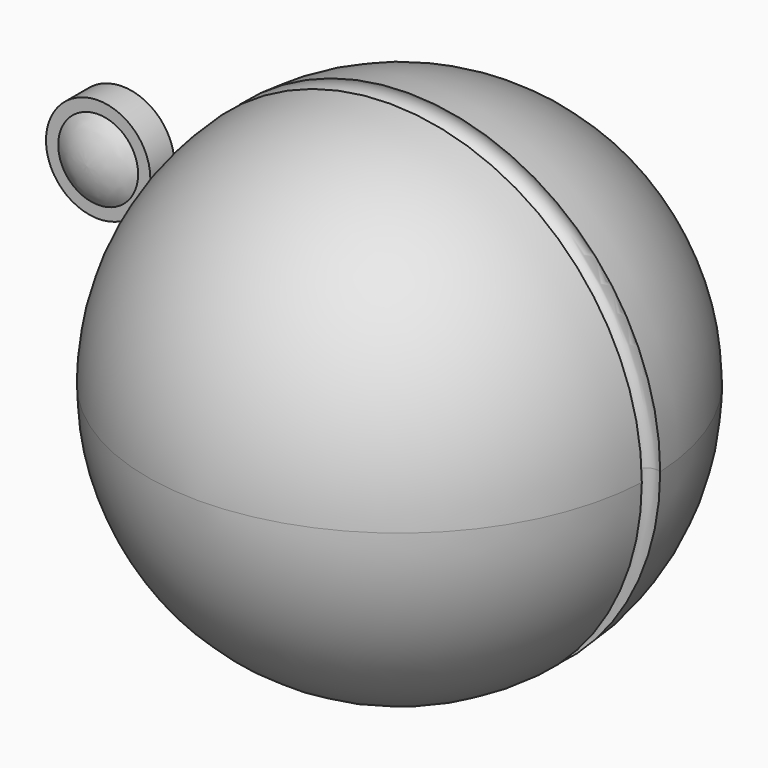
from build123d import *

# Parameters (mm, degrees)
F2_ANGLE  = 180
F5_R      = 7.25
F6_DEPTH  = 25
F8_W      = 26.5384614468
F8_H      = 20.0961548835
F9_DEPTH  = 20.8
F10_R     = 5.5512855598
F11_DEPTH = 2


# Not quite as in the source:
# - a fillet or chamfer that OpenCascade refuses, or shapes differently, is made with other operations: its cross-section is extruded or revolved along the edge and cut away or added


with BuildPart() as f2:
    # F0 (on Top) → F2 (revolve)
    with BuildSketch(Plane.XY):
        with BuildLine():
            Line((0, 30), (0, 35))
            ThreePointArc((0, 35), (-24.1771803229, 25.3073892694), (-34.9635036496, 1.5979400934))
            ThreePointArc((-34.9635036496, 1.5979400934), (-33.2976690142, 1.4681844889), (-32.5, 0))
            ThreePointArc((-32.5, 0), (-33.2976690142, -1.4681844889), (-34.9635036496, -1.5979400934))
            ThreePointArc((-34.9635036496, -1.5979400934), (-24.1771803229, -25.3073892694), (0, -35))
            Line((0, -35), (0, -30))
            ThreePointArc((0, -30), (-30, 0), (0, 30))
        make_face()
    revolve(axis=Axis((0, 0.055314973, 0), (0, -1, 0)), revolution_arc=F2_ANGLE)


with BuildPart() as f3_1:
    # F3: instance of F2
    add(f2.part.mirror(Plane.XY))


with BuildPart() as f6:
    # F5 (on Front) → F6 (new body)
    with BuildSketch(Plane.XZ):
        with Locations((-58.4951840291, 0)):
            Circle(F5_R)
    extrude(amount=-F6_DEPTH)

    # F4 (on Top) → F7 (revolve)
    with BuildSketch(Plane.XY):
        with BuildLine():
            Line((-58.4951840291, 24.5332963728), (-58.4951840291, 27.9332963728))
            ThreePointArc((-58.4951840291, 27.9332963728), (-60.1951840291, 26.2332963728), (-58.4951840291, 24.5332963728))
        make_face()
    revolve(axis=Axis((-58.4951840291, 26.2332963728, 0), (0, -1, 0)))

    # F8 (on Front) → F9 (cut)
    with BuildSketch(Plane.XZ):
        with Locations((-55.8634325862, -0.4141749814)):
            Rectangle(F8_W, F8_H)
    extrude(amount=-F9_DEPTH, mode=Mode.SUBTRACT)

    # F10 (on face) → F11 (join)
    with BuildSketch(Plane.XZ.offset(-20.8)):
        with Locations((-58.4951840291, 0)):
            Circle(F10_R)
    extrude(amount=F11_DEPTH)

    # F12: fillet of radius 8.68 on 1 edges, made by hand

    # F12_s1 → F12_t2 (revolve, cut)
    with BuildSketch(Plane.XY):
        with BuildLine():
            ThreePointArc((-52.9438984693, 20.8), (-55.540277081, 19.3152954738), (-58.4864610535, 18.8))
            Line((-58.4864610535, 18.8), (-52.9438984693, 18.8))
            Line((-52.9438984693, 18.8), (-52.9438984693, 20.8))
        make_face()
    revolve(axis=Axis((-58.4951840291, 18.8, 0), (0, -1, 0)), mode=Mode.SUBTRACT)


solid = Compound([f2.part, f3_1.part, f6.part])
